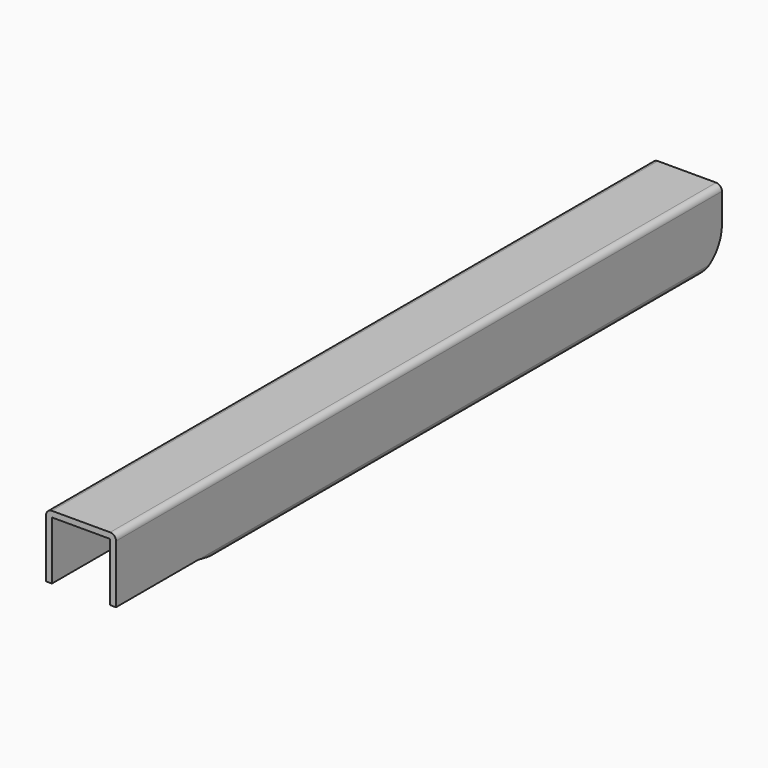
from build123d import *

# Parameters (mm, degrees)
F0_W     = 50
F0_H     = 50
F1_DEPTH = 325
F3_DEPTH = 60.001


# Not quite as in the source:
# - a feature names something its author has since deleted; it is built from what else it names


with BuildPart() as f1:
    # F0 (on Front) → F1 (new body, symmetric)
    with BuildSketch(Plane.XZ):
        with BuildLine():
            Line((-25, -30), (25, -30))
            ThreePointArc((25, -30), (28.5355339059, -28.5355339059), (30, -25))
            Line((30, -25), (30, 25))
            ThreePointArc((30, 25), (28.5355339059, 28.5355339059), (25, 30))
            Line((25, 30), (-25, 30))
            ThreePointArc((-25, 30), (-28.5355339059, 28.5355339059), (-30, 25))
            Line((-30, 25), (-30, -25))
            ThreePointArc((-30, -25), (-28.5355339059, -28.5355339059), (-25, -30))
        make_face()
        Rectangle(F0_W, F0_H, mode=Mode.SUBTRACT)
    extrude(amount=F1_DEPTH, both=True)

    # F2 (on face) → F3 (cut, through all)
    with BuildSketch(Plane.YZ.offset(30)):
        Polygon((-325, -5), (-347.579985857, -5), (-354.4286191463, -50.3063426539), (-215, -50.3063426539), (-215, -30), (-237, -25), (-325, -25), align=None)
        with BuildLine():
            Line((325, -25), (311.5831239518, -25))
            ThreePointArc((311.5831239518, -25), (303.6602540378, -28.7228132327), (295, -30))
            Line((295, -30), (295, -47.2164526592))
            Line((295, -47.2164526592), (357.106402663, -47.2164526592))
            Line((357.106402663, -47.2164526592), (357.106402663, 0))
            Line((357.106402663, 0), (325, 0))
            Line((325, 0), (325, -25))
        make_face()
        with BuildLine():
            ThreePointArc((325, 0), (321.4338203685, -14.1863716546), (311.5831239518, -25))
            Line((311.5831239518, -25), (325, -25))
            Line((325, -25), (325, 0))
        make_face()
    extrude(amount=-F3_DEPTH, mode=Mode.SUBTRACT)


solid = f1.part
